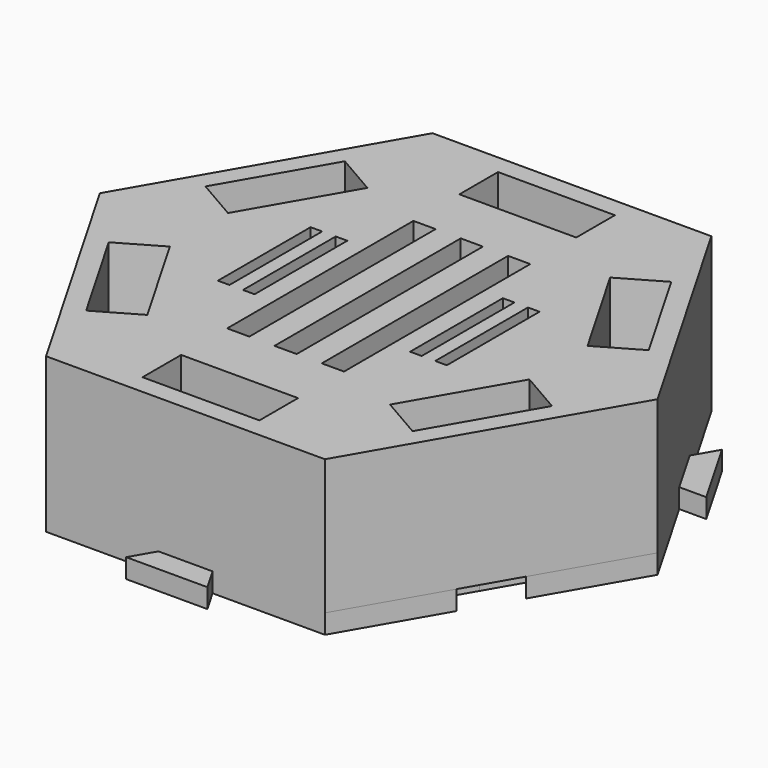
from build123d import *

# Parameters (mm, degrees)
F1_DEPTH        = 2
F3_DEPTH        = 14
F4_W            = 12.1
F4_H            = 5
F5_DEPTH        = 13.5
F6_W            = 2.3
F6_H            = 24.1
F7_DEPTH        = 13.5
F8_W            = 1.2
F8_H            = 12
F9_DEPTH        = 12
F11_DEPTH       = 1
F12_TEXT_SIZE   = 2.6214467109
F12_TEXT_SIZE_2 = 3.0441400304
F12_TEXT_SIZE_3 = 2.1957286217
F13_DEPTH       = 1


# Not quite as in the source:
# - a feature names something its author has since deleted; it is built from what else it names
# - Text() gives the source's letters only with a copy of the font that has no kerning and outlines rounded to 1/6400 em; it was checked with that copy


with BuildPart() as f1:
    # F0 (on Top) → F1 (new body)
    with BuildSketch(Plane.XY):
        Polygon((4.2, -27.4248711306), (2.8, -25), (0, -25), (-2.8, -25), (-4.2, -27.4248711306), (0, -27.4248711306), align=None)
        Polygon((20.2506350946, 14.9248711306), (14.4337567297, 25), (3, 25), (4.5, 22.4019237886), (0, 22.4019237886), (-4.5, 22.4019237886), (-3, 25), (-14.4337567297, 25), (-16.245760443, 21.8615175051), (-20.2506350946, 14.9248711306), (-23.0506350946, 10.0751288694), (-28.8675134595, 0), (-23.1506350946, -9.9019237886), (-21.6506350946, -7.3038475773), (-19.4006350946, -11.2009618943), (-17.1506350946, -15.0980762114), (-20.1506350946, -15.0980762114), (-14.4337567297, -25), (-2.8, -25), (0, -25), (2.8, -25), (14.4337567297, -25), (20.1506350946, -15.0980762114), (17.1506350946, -15.0980762114), (19.4006350946, -11.2009618943), (21.6506350946, -7.3038475773), (23.1506350946, -9.9019237886), (28.8675134595, 0), (23.0506350946, 10.0751288694), align=None)
        Polygon((21.6506350946, 17.3497422612), (20.2506350946, 14.9248711306), (23.0506350946, 10.0751288694), (25.8506350946, 10.0751288694), (23.7506350946, 13.7124355653), align=None)
        Polygon((-23.0506350946, 10.0751288694), (-20.2506350946, 14.9248711306), (-21.6506350946, 17.3497422612), (-23.7506350946, 13.7124355653), (-25.8506350946, 10.0751288694), align=None)
    extrude(amount=F1_DEPTH)

    # F2 (on face) → F3 (join)
    with BuildSketch(Plane.XY.offset(2)):
        Polygon((-28.8675134595, 0), (-14.4337567297, -25), (14.4337567297, -25), (28.8675134595, 0), (14.4337567297, 25), (-14.4337567297, 25), align=None)
    extrude(amount=F3_DEPTH)

    # F4 (on face) → F5 (cut)
    with BuildSketch(Plane.XY.offset(16)):
        with Locations((0, -20.5)):
            Rectangle(F4_W, F4_H)
        Polygon((16.893584287, -16.7394536929), (22.943584287, -6.2605463071), (18.6134572681, -3.7605463071), (12.5634572681, -14.2394536929), align=None)
        Polygon((22.943584287, 6.2605463071), (16.893584287, 16.7394536929), (12.5634572681, 14.2394536929), (18.6134572681, 3.7605463071), align=None)
        with Locations((0, 20.5)):
            Rectangle(F4_W, F4_H)
        Polygon((-16.893584287, 16.7394536929), (-22.943584287, 6.2605463071), (-18.6134572681, 3.7605463071), (-12.5634572681, 14.2394536929), align=None)
        Polygon((-22.943584287, -6.2605463071), (-16.893584287, -16.7394536929), (-12.5634572681, -14.2394536929), (-18.6134572681, -3.7605463071), align=None)
    extrude(amount=-F5_DEPTH, mode=Mode.SUBTRACT)

    # F6 (on face) → F7 (cut)
    with BuildSketch(Plane.XY.offset(16)):
        with Locations((-4.9, 0)):
            Rectangle(F6_W, F6_H)
        Rectangle(F6_W, F6_H)
        with Locations((4.9, 0)):
            Rectangle(F6_W, F6_H)
    extrude(amount=-F7_DEPTH, mode=Mode.SUBTRACT)

    # F8 (on face) → F9 (cut)
    with BuildSketch(Plane.XY.offset(16)):
        with Locations((-8.65, 0)):
            Rectangle(F8_W, F8_H)
        with Locations((-11.25, 0)):
            Rectangle(F8_W, F8_H)
        with Locations((11.25, 0)):
            Rectangle(F8_W, F8_H)
        with Locations((8.65, 0)):
            Rectangle(F8_W, F8_H)
    extrude(amount=-F9_DEPTH, mode=Mode.SUBTRACT)

    # F10 (on face) → F11 (cut)
    with BuildSketch(Plane(origin=(0, 0, 0), x_dir=(1, 0, 0), z_dir=(0, 0, -1))):
        Polygon((-7.5055534995, -13), (7.5055534995, -13), (15.0111069989, 0), (7.5055534995, 13), (-7.5055534995, 13), (-15.0111069989, 0), align=None)
    extrude(amount=-F11_DEPTH, mode=Mode.SUBTRACT)

    # F12 (on face) → F13 (join)
    with BuildSketch(Plane(origin=(0, 0, 1), x_dir=(1, 0, 0), z_dir=(0, 0, -1))):
        with Locations((-10, -5.9833320428)):
            Text('USB / SD / Micro', F12_TEXT_SIZE, font='Open Sans', text_align=(TextAlign.LEFT, TextAlign.BOTTOM))
        with Locations((-5, -1.095890411)):
            Text('720tec', F12_TEXT_SIZE_2, font='Open Sans', font_style=FontStyle.BOLD, text_align=(TextAlign.LEFT, TextAlign.BOTTOM))
        with Locations((-4, 4.095890411)):
            Text('bblasco', F12_TEXT_SIZE_3, font='Open Sans', font_style=FontStyle.BOLDITALIC, text_align=(TextAlign.LEFT, TextAlign.BOTTOM))
    extrude(amount=F13_DEPTH)


solid = f1.part
